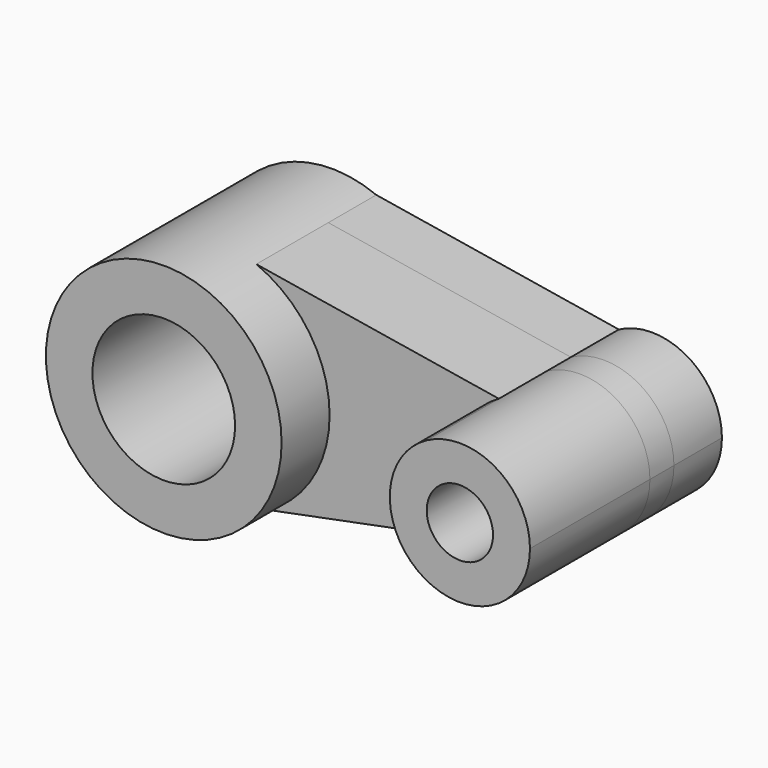
from build123d import *

# Parameters (mm, degrees)
F0_R     = 14.0379672149
F2_DEPTH = 25.4
F0_R_2   = 30.2035472703
F4_DEPTH = 63.5
F5_DEPTH = 38.1
F6_DEPTH = 12.7
F7_DEPTH = 63.5


with BuildPart() as f2:
    # F0 (on Front) → F2 (new body)
    with BuildSketch(Plane.XZ):
        with BuildLine():
            ThreePointArc((95.2809938719, 31.1565697193), (80.867987619, 56.6041793229), (51.6312028736, 57.3294389535))
            ThreePointArc((51.6312028736, 57.3294389535), (35.965029482, 29.8828413836), (53.9277169218, 3.88117669))
            ThreePointArc((53.9277169218, 3.88117669), (81.9463228304, 6.3874327773), (95.2809938719, 31.1565697193))
        make_face()
        with Locations((65.6093358994, 31.1565697193)):
            Circle(F0_R, mode=Mode.SUBTRACT)
    extrude(amount=F2_DEPTH)


with BuildPart() as f2b:
    # F0 (on Front) → F2, piece 2 (new body)
    with BuildSketch(Plane.XZ):
        with BuildLine():
            ThreePointArc((-45.9266097252, -15.8601469004), (-26.9891091759, 2.4701327863), (-20.0295753742, 27.890458703))
            ThreePointArc((-20.0295753742, 27.890458703), (-28.508832265, 55.7187391388), (-51.0652040106, 74.0904860103))
            ThreePointArc((-51.0652040106, 74.0904860103), (-119.7579132685, 25.0441972115), (-45.9266097252, -15.8601469004))
        make_face()
        with Locations((-69.934360683, 27.890458703)):
            Circle(F0_R_2, mode=Mode.SUBTRACT)
    extrude(amount=F2_DEPTH)

    # F4 (add): a face of the model
    f4_faces = [f2b.faces().sort_by_distance(p)[0] for p in [
        (-93.2630699006, -25.4, 70.4036103104),
    ]]
    extrude(f4_faces, amount=F4_DEPTH)


with BuildPart() as f2c:
    # F1 (on face) → F2, piece 3 (new body)
    with BuildSketch(Plane.XZ):
        with BuildLine():
            Line((51.6312028736, 57.3294389535), (-51.0652040106, 74.0904860103))
            ThreePointArc((-51.0652040106, 74.0904860103), (-28.508832265, 55.7187391388), (-20.0295753742, 27.890458703))
            ThreePointArc((-20.0295753742, 27.890458703), (-26.9891091759, 2.4701327863), (-45.9266097252, -15.8601469004))
            Line((-45.9266097252, -15.8601469004), (53.9277169218, 3.88117669))
            ThreePointArc((53.9277169218, 3.88117669), (35.965029482, 29.8828413836), (51.6312028736, 57.3294389535))
        make_face()
    extrude(amount=F2_DEPTH)


with BuildPart() as f5:
    # F5 (new): a face of the model
    f5_faces = [f2c.part.faces().sort_by_distance(p)[0] for p in [
        (4.6663814886, -25.4, 29.8185425635),
    ]]
    extrude(f5_faces, amount=F5_DEPTH)


with BuildPart() as f6:
    # F6 (new): a face of the model
    f6_faces = [f2.part.faces().sort_by_distance(p)[0] for p in [
        (76.9605487971, -25.4, 57.6604981338),
    ]]
    extrude(f6_faces, amount=F6_DEPTH)


with BuildPart() as f7:
    # F7 (new): a face of the model
    f7_faces = [f6.part.faces().sort_by_distance(p)[0] for p in [
        (76.9605487971, -38.1, 57.6604981338),
    ]]
    extrude(f7_faces, amount=F7_DEPTH)


solid = Compound([f2.part, f2b.part, f2c.part, f5.part, f6.part, f7.part])
